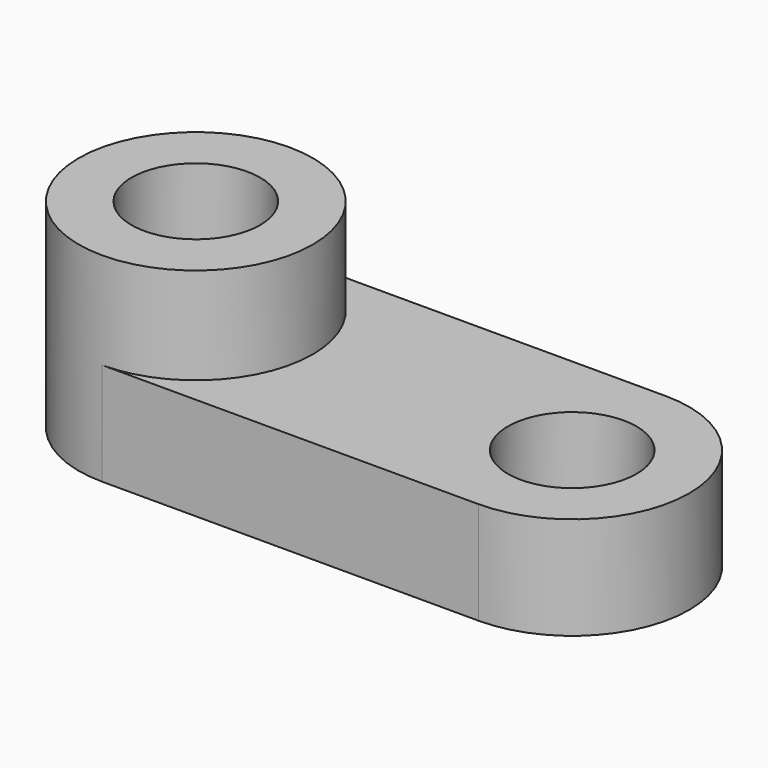
from build123d import *

# Parameters (mm, degrees)
F0_R     = 15.9205
F1_DEPTH = 25.4
F2_DEPTH = 49.318


# Not quite as in the source:
# - a feature names something its author has since deleted; it is built from what else it names


with BuildPart() as f1:
    # F0 (on Top) → F1 (new body)
    with BuildSketch(Plane.XY):
        with BuildLine():
            Line((-49.2564179003, -28.975), (43.9025820997, -28.975))
            ThreePointArc((43.9025820997, -28.975), (72.8775820997, 0), (43.9025820997, 28.975))
            Line((43.9025820997, 28.975), (-49.2564179003, 28.975))
            ThreePointArc((-49.2564179003, 28.975), (-28.7679989154, 20.4884189849), (-20.2814179003, 0))
            ThreePointArc((-20.2814179003, 0), (-28.7679989154, -20.4884189849), (-49.2564179003, -28.975))
        make_face()
        with Locations((43.9025820997, 0)):
            Circle(F0_R, mode=Mode.SUBTRACT)
        with BuildLine():
            ThreePointArc((-49.2564179003, 28.975), (-78.2314179003, 0), (-49.2564179003, -28.975))
            ThreePointArc((-49.2564179003, -28.975), (-28.7679989154, -20.4884189849), (-20.2814179003, 0))
            ThreePointArc((-20.2814179003, 0), (-28.7679989154, 20.4884189849), (-49.2564179003, 28.975))
        make_face()
        with Locations((-49.2564179003, 0)):
            Circle(F0_R, mode=Mode.SUBTRACT)
    extrude(amount=F1_DEPTH)

    # F0 (on Top) → F2 (join)
    with BuildSketch(Plane.XY):
        with BuildLine():
            ThreePointArc((-49.2564179003, 28.975), (-78.2314179003, 0), (-49.2564179003, -28.975))
            ThreePointArc((-49.2564179003, -28.975), (-28.7679989154, -20.4884189849), (-20.2814179003, 0))
            ThreePointArc((-20.2814179003, 0), (-28.7679989154, 20.4884189849), (-49.2564179003, 28.975))
        make_face()
        with Locations((-49.2564179003, 0)):
            Circle(F0_R, mode=Mode.SUBTRACT)
    extrude(amount=F2_DEPTH)


solid = f1.part
